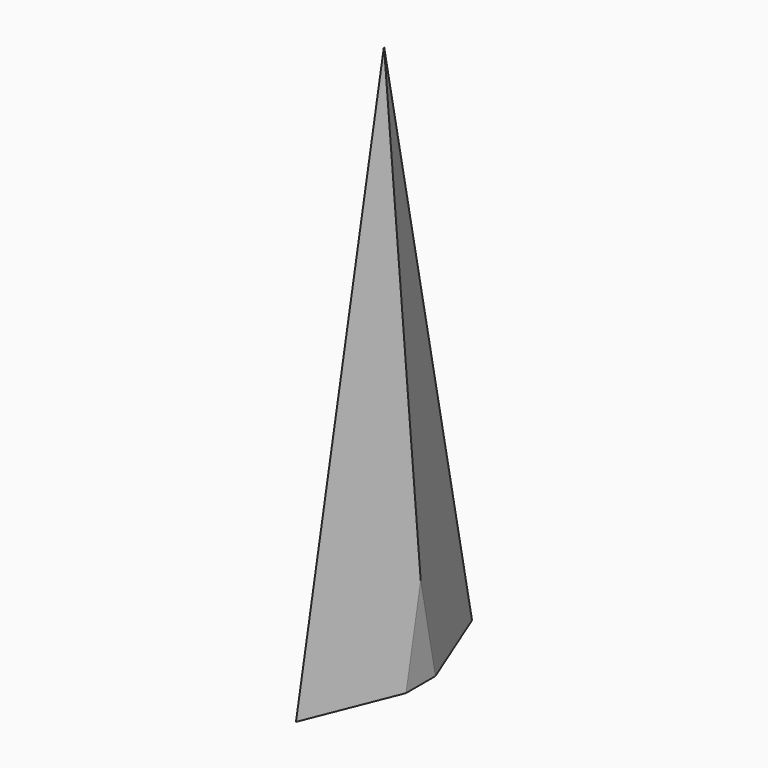
from build123d import *

# Parameters (mm, degrees)
F0_W        = 20
F0_H        = 60
F1_DEPTH    = 150
F2_D        = 6
F2_DEPTH    = 50
F2_TIP      = 1.8025818571
F3_SIZE2    = 29.99999
F3_SIZE     = 149.99999
F3_2_SIZE2  = 29.99999
F3_2_SIZE   = 149.99999
F4_T1_DEPTH = 407.0708695577
F4_T3_DEPTH = 407.0708695577


# Not quite as in the source:
# - a fillet or chamfer that OpenCascade refuses, or shapes differently, is made with other operations: its cross-section is extruded or revolved along the edge and cut away or added
# - a fillet or chamfer is up to 0.001 mm smaller than in the source, because OpenCascade refuses the exact size


with BuildPart() as f1:
    # F0 (on Top) → F1 (new body)
    with BuildSketch(Plane.XY):
        Rectangle(F0_W, F0_H)
    extrude(amount=F1_DEPTH)

    # F2
    with Locations(Plane(origin=(0, 0, 0), x_dir=(1, 0, 0), z_dir=(0, 0, -1))):
        with Locations((0, -10), (0, 0), (0, 10)):
            Hole(F2_D / 2, depth=F2_DEPTH)
            with Locations((0, 0, -(F2_DEPTH + F2_TIP / 2))):  # 118° drill point
                Cone(0, F2_D / 2, F2_TIP, mode=Mode.SUBTRACT)

    # F3 (size 150 and 30 in the source; OpenCascade refuses exactly that, so slightly less here)
    f3_edges = [f1.edges().sort_by_distance(p)[0] for p in [
        (0, -30, 150),
    ]]
    f3_side = f1.faces().sort_by_distance((0, -30, 75))[0]
    chamfer(f3_edges, length=F3_SIZE, length2=F3_SIZE2, reference=f3_side)

    # F3#2 (size 150 and 30 in the source; OpenCascade refuses exactly that, so slightly less here)
    f3_2_edges = [f1.edges().sort_by_distance(p)[0] for p in [
        (0, 30, 150),
    ]]
    f3_2_side = f1.faces().sort_by_distance((0, 30, 75))[0]
    chamfer(f3_2_edges, length=F3_2_SIZE, length2=F3_2_SIZE2, reference=f3_2_side)

    # F4: chamfer of 24.5 x 10 on 4 edges, made by hand

    # F4_s2 → F4_t1 (cut)
    with BuildSketch(Plane(origin=(0, -38.5287100353, -192.6436015479), x_dir=(1, 0, 0), z_dir=(0, 0.1961160849, 0.9805806857))):
        Polygon((0, -29.4174225336), (10, -4.9174225336), (10, -29.4174225336), align=None)
        Polygon((-10, -4.9174225336), (0, -29.4174225336), (-10, -29.4174225336), align=None)
    extrude(amount=F4_T1_DEPTH, mode=Mode.SUBTRACT)

    # F4_s4 → F4_t3 (cut)
    with BuildSketch(Plane(origin=(0, 38.5287100353, -192.6436015479), x_dir=(1, 0, 0), z_dir=(0, -0.1961160849, 0.9805806857))):
        Polygon((0, 29.4174225336), (10, 4.9174225336), (10, 29.4174225336), align=None)
        Polygon((-10, 4.9174225336), (0, 29.4174225336), (-10, 29.4174225336), align=None)
    extrude(amount=F4_T3_DEPTH, mode=Mode.SUBTRACT)


solid = f1.part
